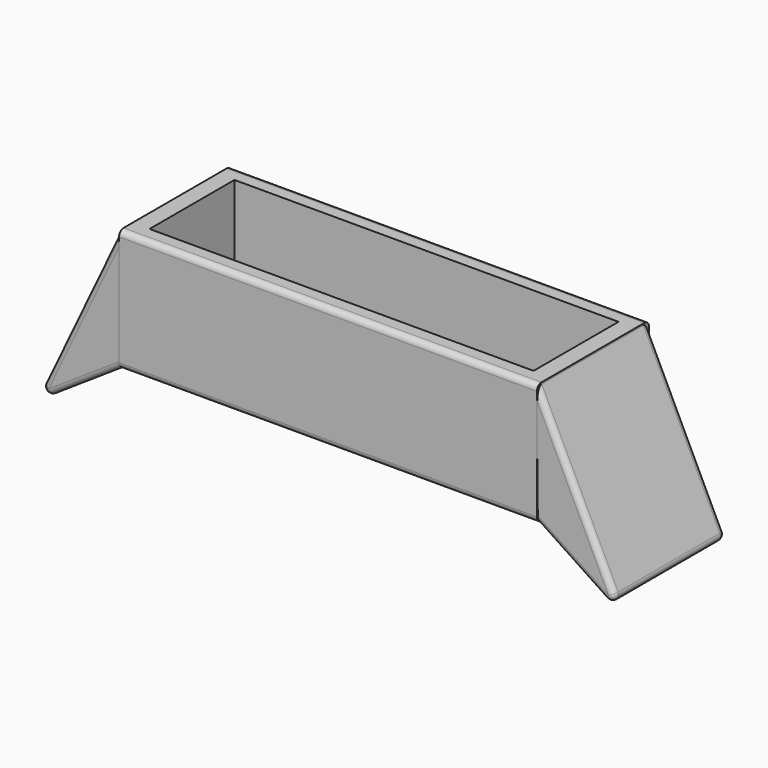
from build123d import *

# Parameters (mm, degrees)
F0_W          = 74
F0_H          = 24.8
F1_DEPTH      = 21.6
F2_DEPTH      = 3
F4_DEPTH      = 13.5
F4_DEPTH_BACK = 11
F5_R          = 1
F6_R          = 1
F7_R          = 1
F8_R          = 1
F9_R          = 1
F10_T1_DEPTH  = 22.5
F10_T6_DEPTH  = 1
F10_T12_DEPTH = 1
F10_T18_DEPTH = 33.6002504657
F10_T23_DEPTH = 33.6002504657
F11_T1_DEPTH  = 22.5
F11_T6_DEPTH  = 1
F11_T12_DEPTH = 1
F11_T18_DEPTH = 33.7248520463
F11_T23_DEPTH = 33.7248520463
F12_R         = 1
F13_R         = 1


# Not quite as in the source:
# - a fillet or chamfer that OpenCascade refuses, or shapes differently, is made with other operations: its cross-section is extruded or revolved along the edge and cut away or added


with BuildPart() as f1:
    # F0 (on Top) → F1 (new body)
    with BuildSketch(Plane.XY):
        with Locations((3.0410322249, 1.3384381361)):
            Rectangle(F0_W, F0_H)
        Polygon((-30.9589677751, -8.0615618639), (-30.9589677751, 10.7384381361), (3.0410322249, 10.7384381361), (37.0410322249, 10.7384381361), (37.0410322249, -8.0615618639), align=None, mode=Mode.SUBTRACT)
    extrude(amount=F1_DEPTH)

    # F0 (on Top) → F2 (join)
    with BuildSketch(Plane.XY):
        Polygon((3.0410322249, 10.7384381361), (-30.9589677751, 10.7384381361), (-30.9589677751, -8.0615618639), (37.0410322249, -8.0615618639), (37.0410322249, 10.7384381361), align=None)
    extrude(amount=F2_DEPTH)

    # F3 (on Front) → F4 (join, two sides)
    with BuildSketch(Plane.XZ) as f4_sk:
        Polygon((-33.8997356594, 21.5996019542), (-48.8997356594, -10), (-33.8997356594, 0), align=None)
        Polygon((39.9138331413, 21.5681958944), (40.1588790119, 0), (55.1588790119, -10), align=None)
    extrude(amount=-F4_DEPTH)
    extrude(f4_sk.sketch, amount=F4_DEPTH_BACK)

    # F5
    f5_edges = [f1.edges().sort_by_distance(p)[0] for p in [
        (3.041032, -11.061562, 0),
    ]]
    fillet(f5_edges, radius=F5_R)

    # F6
    f6_edges = [f1.edges().sort_by_distance(p)[0] for p in [
        (-40.908821, -11, -4.672724),
    ]]
    fillet(f6_edges, radius=F6_R)

    # F7
    f7_edges = [f1.edges().sort_by_distance(p)[0] for p in [
        (47.658879, -11, -5),
    ]]
    fillet(f7_edges, radius=F7_R)

    # F8
    f8_edges = [f1.edges().sort_by_distance(p)[0] for p in [
        (3.041032, 13.738438, 0),
    ]]
    fillet(f8_edges, radius=F8_R)

    # F9
    f9_edges = [f1.edges().sort_by_distance(p)[0] for p in [
        (-41.135805, 13.5, -4.824046),
        (47.658879, 13.5, -5),
    ]]
    fillet(f9_edges, radius=F9_R)

    # F10: fillet of radius 1 on 1 edges, made by hand

    # F10_s2 → F10_t1 (cut)
    with BuildSketch(Plane.XZ.offset(-12.5)):
        with BuildLine():
            ThreePointArc((53.5655977195, -6.7007632263), (53.3217359927, -7.8898447489), (52.1104042723, -7.967683507))
            Line((52.1104042723, -7.967683507), (55.1588790119, -10))
            Line((55.1588790119, -10), (53.5655977195, -6.7007632263))
        make_face()
    extrude(amount=F10_T1_DEPTH, mode=Mode.SUBTRACT)


with BuildPart() as f10_tool4:
    # F10_s5 → F10_t6 (new body)
    with BuildSketch(Plane.XZ.offset(-12.5)):
        Polygon((52.6651044685, -7.1356332126), (52.1104042723, -7.967683507), (55.1588790119, -10), (53.5655977195, -6.7007632263), align=None)
    extrude(amount=-F10_T6_DEPTH)

    # F10_s7 → F10_t8 (revolve, cut)
    with BuildSketch(Plane(origin=(52.6651044685, 12.5, -7.1356332126), x_dir=(-0.6566315242, 0, 0.7542115363), z_dir=(-0.7542115363, 0, -0.6566315242))):
        with BuildLine():
            ThreePointArc((0, -1), (1, 0), (0, 1))
            Line((0, 1), (0, -1))
        make_face()
    revolve(axis=Axis((52.6651044685, 12.5, -7.1356332126), (0, 1, 0)), mode=Mode.SUBTRACT)


with BuildPart() as f1_1:
    add(f1.part)

    # F10_t3: cut F10_tool4
    add(f10_tool4.part, mode=Mode.SUBTRACT)


with BuildPart() as f10_tool10:
    # F10_s11 → F10_t12 (new body)
    with BuildSketch(Plane.XZ.offset(10)):
        Polygon((52.6651044685, -7.1356332126), (53.5655977195, -6.7007632263), (55.1588790119, -10), (52.1104042723, -7.967683507), align=None)
    extrude(amount=F10_T12_DEPTH)

    # F10_s13 → F10_t14 (revolve, cut)
    with BuildSketch(Plane(origin=(52.6651044685, -10, -7.1356332126), x_dir=(-0.6566315242, 0, 0.7542115363), z_dir=(0.7542115363, 0, 0.6566315242))):
        with BuildLine():
            ThreePointArc((0, -1), (1, 0), (0, 1))
            Line((0, 1), (0, -1))
        make_face()
    revolve(axis=Axis((52.6651044685, -10, -7.1356332126), (0, -1, 0)), mode=Mode.SUBTRACT)


with BuildPart() as f1_2:
    add(f1_1.part)

    # F10_t9: cut F10_tool10
    add(f10_tool10.part, mode=Mode.SUBTRACT)


with BuildPart() as f10_tool16:
    # F10_s17 → F10_t18 (new body)
    with BuildSketch(Plane(origin=(12.7538942726, 0, -26.4097226228), x_dir=(0, 1, 0), z_dir=(-0.4348699863, 0, 0.9004932509))):
        with BuildLine():
            ThreePointArc((12.5, -45.3214984167), (13.2071067812, -45.0286051978), (13.5, -44.3214984167))
            Line((13.5, -44.3214984167), (13.5, -45.3214984167))
            Line((13.5, -45.3214984167), (12.5, -45.3214984167))
        make_face()
    extrude(amount=F10_T18_DEPTH)

    split(bisect_by=Plane.YZ.offset(40.0410322249), keep=Keep.TOP)


with BuildPart() as f1_3:
    add(f1_2.part)

    # F10_t15: cut F10_tool16
    add(f10_tool16.part, mode=Mode.SUBTRACT)


with BuildPart() as f10_tool21:
    # F10_s22 → F10_t23 (new body)
    with BuildSketch(Plane(origin=(12.7538942726, 0, -26.4097226228), x_dir=(0, 1, 0), z_dir=(-0.4348699863, 0, 0.9004932509))):
        with BuildLine():
            ThreePointArc((-10, -45.3214984167), (-10.7071067812, -45.0286051978), (-11, -44.3214984167))
            Line((-11, -44.3214984167), (-11, -45.3214984167))
            Line((-11, -45.3214984167), (-10, -45.3214984167))
        make_face()
    extrude(amount=F10_T23_DEPTH)

    split(bisect_by=Plane.YZ.offset(40.0410322249), keep=Keep.TOP)


with BuildPart() as f1_4:
    add(f1_3.part)

    # F10_t20: cut F10_tool21
    add(f10_tool21.part, mode=Mode.SUBTRACT)

    # F11: fillet of radius 1 on 1 edges, made by hand

    # F11_s2 → F11_t1 (cut)
    with BuildSketch(Plane.XZ.offset(-12.5)):
        with BuildLine():
            ThreePointArc((-45.890970827, -7.9941567784), (-47.0997726727, -7.918513142), (-47.3490572007, -6.7332785298))
            Line((-47.3490572007, -6.7332785298), (-48.8997356594, -10))
            Line((-48.8997356594, -10), (-45.890970827, -7.9941567784))
        make_face()
    extrude(amount=F11_T1_DEPTH, mode=Mode.SUBTRACT)


with BuildPart() as f11_tool4:
    # F11_s5 → F11_t6 (new body)
    with BuildSketch(Plane.XZ.offset(-12.5)):
        Polygon((-46.4456710232, -7.1621064841), (-47.3490572007, -6.7332785298), (-48.8997356594, -10), (-45.890970827, -7.9941567784), align=None)
    extrude(amount=-F11_T6_DEPTH)

    # F11_s7 → F11_t8 (revolve, cut)
    with BuildSketch(Plane(origin=(-46.4456710232, 12.5, -7.1621064841), x_dir=(0.6541016495, 0, 0.7564066579), z_dir=(-0.7564066579, 0, 0.6541016495))):
        with BuildLine():
            ThreePointArc((0, -1), (1, 0), (0, 1))
            Line((0, 1), (0, -1))
        make_face()
    revolve(axis=Axis((-46.4456710232, 12.5, -7.1621064841), (0, 1, 0)), mode=Mode.SUBTRACT)


with BuildPart() as f1_5:
    add(f1_4.part)

    # F11_t3: cut F11_tool4
    add(f11_tool4.part, mode=Mode.SUBTRACT)


with BuildPart() as f11_tool10:
    # F11_s11 → F11_t12 (new body)
    with BuildSketch(Plane.XZ.offset(10)):
        Polygon((-46.4456710232, -7.1621064841), (-47.3490572007, -6.7332785298), (-48.8997356594, -10), (-45.890970827, -7.9941567784), align=None)
    extrude(amount=F11_T12_DEPTH)

    # F11_s13 → F11_t14 (revolve, cut)
    with BuildSketch(Plane(origin=(-46.4456710232, -10, -7.1621064841), x_dir=(0.6541016495, 0, 0.7564066579), z_dir=(0.7564066579, 0, -0.6541016495))):
        with BuildLine():
            ThreePointArc((0, -1), (1, 0), (0, 1))
            Line((0, 1), (0, -1))
        make_face()
    revolve(axis=Axis((-46.4456710232, -10, -7.1621064841), (0, -1, 0)), mode=Mode.SUBTRACT)


with BuildPart() as f1_6:
    add(f1_5.part)

    # F11_t9: cut F11_tool10
    add(f11_tool10.part, mode=Mode.SUBTRACT)


with BuildPart() as f11_tool16:
    # F11_s17 → F11_t18 (new body)
    with BuildSketch(Plane(origin=(3.1465259538, 0, 6.6285978453), x_dir=(0, 1, 0), z_dir=(-0.4288279543, 0, -0.9033861775))):
        with BuildLine():
            ThreePointArc((12.5, -39.8870657335), (13.2071067812, -39.5941725147), (13.5, -38.8870657335))
            Line((13.5, -38.8870657335), (13.5, -39.8870657335))
            Line((13.5, -39.8870657335), (12.5, -39.8870657335))
        make_face()
    extrude(amount=F11_T18_DEPTH)

    split(bisect_by=Plane.YZ.offset(-33.9589677751), keep=Keep.BOTTOM)


with BuildPart() as f1_7:
    add(f1_6.part)

    # F11_t15: cut F11_tool16
    add(f11_tool16.part, mode=Mode.SUBTRACT)


with BuildPart() as f11_tool21:
    # F11_s22 → F11_t23 (new body)
    with BuildSketch(Plane(origin=(3.1465259538, 0, 6.6285978453), x_dir=(0, 1, 0), z_dir=(-0.4288279543, 0, -0.9033861775))):
        with BuildLine():
            ThreePointArc((-10, -39.8870657335), (-10.7071067812, -39.5941725147), (-11, -38.8870657335))
            Line((-11, -38.8870657335), (-11, -39.8870657335))
            Line((-11, -39.8870657335), (-10, -39.8870657335))
        make_face()
    extrude(amount=F11_T23_DEPTH)

    split(bisect_by=Plane.YZ.offset(-33.9589677751), keep=Keep.BOTTOM)


with BuildPart() as f1_8:
    add(f1_7.part)

    # F11_t20: cut F11_tool21
    add(f11_tool21.part, mode=Mode.SUBTRACT)

    # F12
    f12_edges = [f1_8.edges().sort_by_distance(p)[0] for p in [
        (3.041032, 13.738438, 21.6),
    ]]
    fillet(f12_edges, radius=F12_R)

    # F13
    f13_edges = [f1_8.edges().sort_by_distance(p)[0] for p in [
        (3.041032, -11.061562, 21.6),
    ]]
    fillet(f13_edges, radius=F13_R)


solid = f1_8.part
